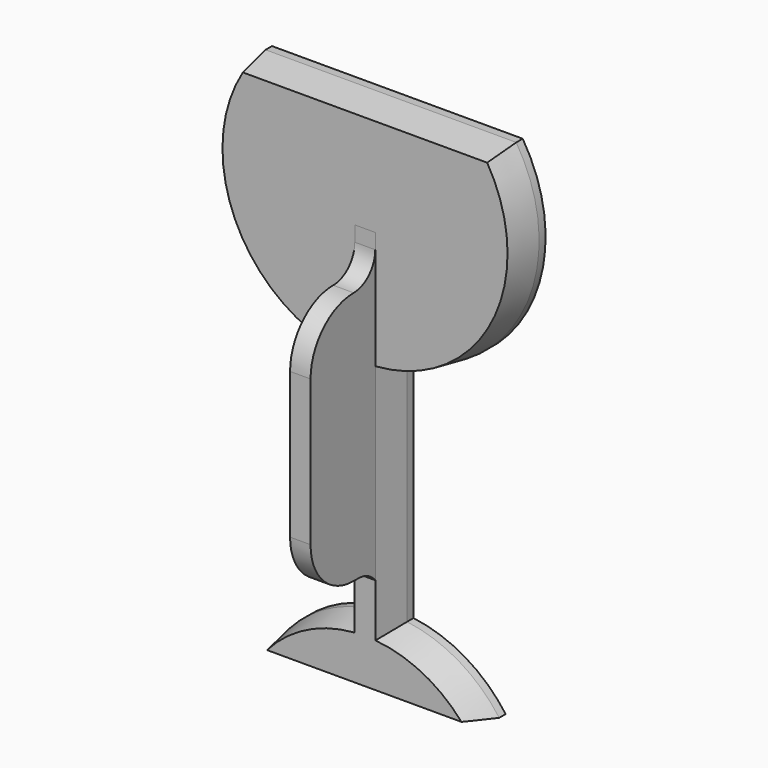
from build123d import *

# Parameters (mm, degrees)
F1_DEPTH               = 1.5
F2_DEPTH               = 6
DRAFT_F2_DRAFTED_ANGLE = 10
F4_DEPTH               = 1.9
F5_R                   = 10
F6_R                   = 10
F7_T1_DEPTH            = 3.8


# Not quite as in the source:
# - a fillet or chamfer that OpenCascade refuses, or shapes differently, is made with other operations: its cross-section is extruded or revolved along the edge and cut away or added
# - an extrude with a draft is written as a straight extrude whose walls are then drafted


with BuildPart() as f1:
    # F0 (on Front) → F1 (new body)
    with BuildSketch(Plane.XZ):
        with BuildLine():
            Line((23.2547415401, 68.7697125971), (-23.2547415401, 68.7697125971))
            ThreePointArc((-23.2547415401, 68.7697125971), (-24.7716760997, 42.1488054955), (-2.9999993183, 26.7550445677))
            Line((-2.9999993183, 26.7550445677), (-2.9999993183, -16.0730433406))
            ThreePointArc((-2.9999993183, -16.0730433406), (-12.7566323722, -19.3253470126), (-20.3783884645, -26.2302874029))
            Line((-20.3783884645, -26.2302874029), (20.0954551433, -26.2302874029))
            ThreePointArc((20.0954551433, -26.2302874029), (12.5965188858, -19.3976025975), (3.0000006817, -16.1072431942))
            Line((3.0000006817, -16.1072431942), (2.9999993183, 26.7550445677))
            ThreePointArc((2.9999993183, 26.7550445677), (24.7716760997, 42.1488054955), (23.2547415401, 68.7697125971))
        make_face()
    extrude(amount=F1_DEPTH)


with BuildPart() as f2_drafted:
    # F2 (new): a face of the model
    f2_faces = [f1.part.faces().sort_by_distance(p)[0] for p in [
        (-0.016488293, -1.5, 36.8691660615),
    ]]
    extrude(f2_faces, amount=F2_DEPTH)

    # draft_F2_drafted
    draft_f2_drafted_walls = [f2_drafted.faces().sort_by_distance(p)[0] for p in [
        (-12.7566323722, -5.5, -19.3253470126),
        (-0.1414666606, -5.5, -26.2302874029),
        (12.5965188858, -5.5, -19.3976025975),
        (3, -5.5, 5.3239006868),
        (24.7716760997, -5.5, 42.1488054955),
        (0, -5.5, 68.7697125971),
        (-24.7716760997, -5.5, 42.1488054955),
        (-2.9999993183, -5.5, 5.3410006136),
    ]]
    draft(draft_f2_drafted_walls, neutral_plane=Plane(origin=(-0.016488293, -1.5, 36.8691660615), x_dir=(1, 0, 0), z_dir=(0, -1, 0)), angle=DRAFT_F2_DRAFTED_ANGLE)


with BuildPart() as f1_1:
    add(f1.part)

    # join_F2_drafted: union F2_drafted
    add(f2_drafted.part)

    # F3 (on Right) → F4 (join, symmetric)
    with BuildSketch(Plane.YZ):
        Polygon((-22.5, -5.3319875151), (-7.5, -5.3319875151), (-7.5000008941, -7.2377305478), (-2.5000008941, -7.2377305478), (-2.5000008941, 49.5622694522), (-7.5000008941, 49.5622694522), (-7.5000008941, 41.7308285832), (-22.5000008941, 41.7308285832), align=None)
    extrude(amount=F4_DEPTH, both=True)

    # F5
    f5_edges = [f1_1.edges().sort_by_distance(p)[0] for p in [
        (0, -22.5, -5.331988),
    ]]
    fillet(f5_edges, radius=F5_R)

    # F6
    f6_edges = [f1_1.edges().sort_by_distance(p)[0] for p in [
        (0, -22.500001, 41.730829),
    ]]
    fillet(f6_edges, radius=F6_R)

    # F7: fillet of radius 5 on 2 edges, made by hand

    # F7_s2 → F7_t1 (join)
    with BuildSketch(Plane.YZ.offset(-1.9)):
        with BuildLine():
            ThreePointArc((-11.4275413229, -5.3319875151), (-9.2448004813, -5.8335830848), (-7.5000008941, -7.2377305478))
            Line((-7.5000008941, -7.2377305478), (-7.5, -5.3319875151))
            Line((-7.5, -5.3319875151), (-11.4275413229, -5.3319875151))
        make_face()
        with BuildLine():
            ThreePointArc((-12.5000008307, 41.7308285832), (-8.9644669657, 43.1952946997), (-7.5000008941, 46.7308285832))
            Line((-7.5000008941, 46.7308285832), (-7.0000008941, 46.7308285832))
            Line((-7.0000008941, 46.7308285832), (-7.0000008941, 41.2308285832))
            Line((-7.0000008941, 41.2308285832), (-12.5000008244, 41.2308285832))
            Line((-12.5000008244, 41.2308285832), (-12.5000008307, 41.7308285832))
        make_face()
    extrude(amount=F7_T1_DEPTH)


solid = f1_1.part
